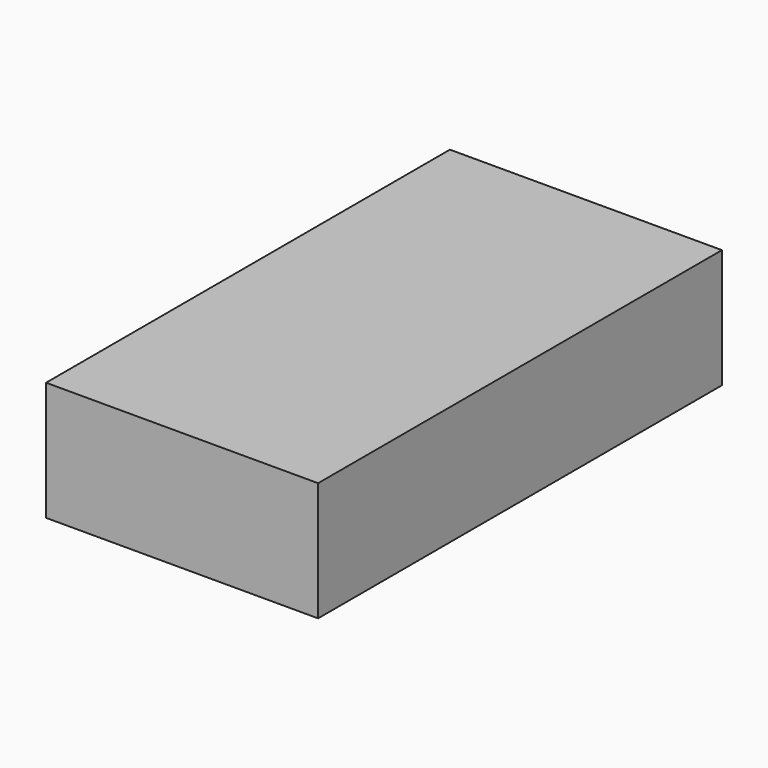
from build123d import *

# Parameters (mm, degrees)
F0_W     = 17.78
F0_H     = 37.338
F0_R     = 1.143
F1_DEPTH = 1.5875
F3_W     = 22.86
F3_H     = 42.418
F3_W_2   = 17.78
F3_H_2   = 37.338
F4_DEPTH = 10


# Not quite as in the source:
# - a feature names something its author has since deleted; it is built from what else it names


with BuildPart() as f1:
    # F0 (on Top) → F1 (new body)
    with BuildSketch(Plane.XY):
        with Locations((-8.89, 18.669)):
            Rectangle(F0_W, F0_H)
        with Locations((-8.89, 9.652)):
            Circle(F0_R, mode=Mode.SUBTRACT)
        with Locations((-15.875, 35.56)):
            Circle(F0_R, mode=Mode.SUBTRACT)
        with Locations((-1.905, 35.56)):
            Circle(F0_R, mode=Mode.SUBTRACT)
    extrude(amount=F1_DEPTH)


with BuildPart() as f4:
    # F3 (on offset) → F4 (new body)
    with BuildSketch(Plane(origin=(0, 0, 2.54), x_dir=(1, 0, 0), z_dir=(0, 0, -1))):
        with Locations((-8.89, -18.669)):
            Rectangle(F3_W, F3_H)
        with Locations((-8.89, -18.669)):
            Rectangle(F3_W_2, F3_H_2, mode=Mode.SUBTRACT)
        with Locations((-8.89, -18.669)):
            Rectangle(F3_W_2, F3_H_2)
    extrude(amount=F4_DEPTH)

    # F5: cut F1
    add(f1.part, mode=Mode.SUBTRACT)


solid = Compound([f1.part, f4.part])
